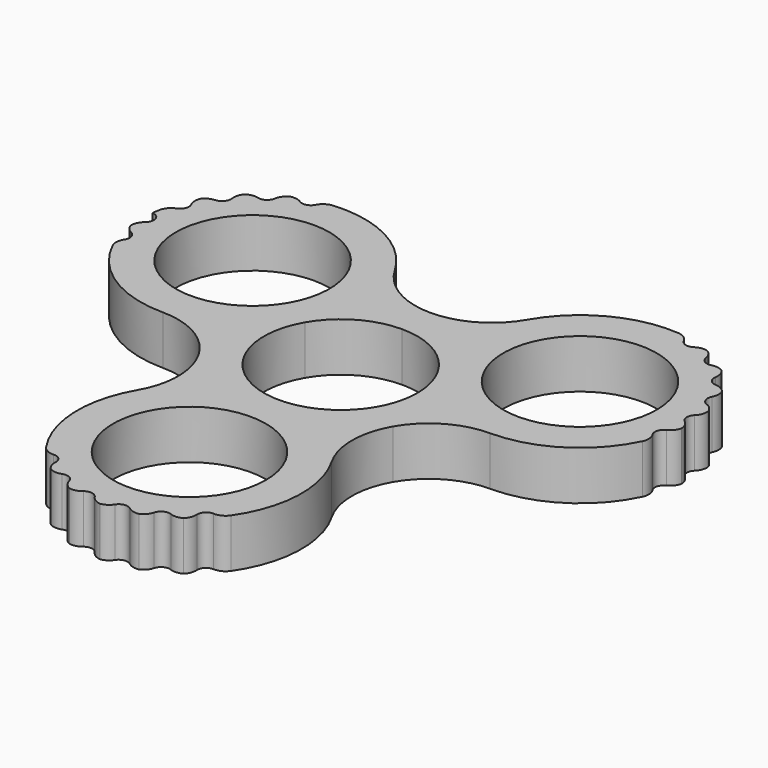
from build123d import *

# Parameters (mm, degrees)
F0_R        = 10.9363137741
F1_DEPTH    = 7.00024
F3_DEPTH    = 7.00124
F4_T1_DEPTH = 14.8104657411
F4_T3_DEPTH = 14.8131793158


# Not quite as in the source:
# - a fillet or chamfer that OpenCascade refuses, or shapes differently, is made with other operations: its cross-section is extruded or revolved along the edge and cut away or added


with BuildPart() as f1:
    # F0 (on Top) → F1 (new body)
    with BuildSketch(Plane.XY):
        with BuildLine():
            ThreePointArc((0, 10.99058), (5.49529, 9.5181214823), (9.5181214823, 5.49529))
            Line((9.5181214823, 5.49529), (13.9175305336, 8.03529))
            ThreePointArc((13.9175305336, 8.03529), (17.9403620159, 23.0487014823), (32.9537734982, 19.02587))
            Line((32.9537734982, 19.02587), (37.3531825494, 21.56587))
            ThreePointArc((37.3531825494, 21.56587), (23.4356520159, 29.60116), (9.5181214823, 21.56587))
            ThreePointArc((9.5181214823, 21.56587), (5.49529, 17.5430385177), (0, 16.07058))
            Line((0, 16.07058), (0, 10.99058))
        make_face()
        with BuildLine():
            Line((13.9175305336, 8.03529), (9.5181214823, 5.49529))
            ThreePointArc((9.5181214823, 5.49529), (10.99058, 0), (9.5181214823, -5.49529))
            Line((9.5181214823, -5.49529), (13.9175305336, -8.03529))
            ThreePointArc((13.9175305336, -8.03529), (17.9403620159, -4.0124585177), (23.4356520159, -2.54))
            ThreePointArc((23.4356520159, -2.54), (37.3531825494, 5.49529), (37.3531825494, 21.56587))
            Line((37.3531825494, 21.56587), (32.9537734982, 19.02587))
            ThreePointArc((32.9537734982, 19.02587), (28.9309420159, 4.0124585177), (13.9175305336, 8.03529))
        make_face()
        with BuildLine():
            Line((13.9175305336, -8.03529), (9.5181214823, -5.49529))
            ThreePointArc((9.5181214823, -5.49529), (0, -10.99058), (-9.5181214823, -5.49529))
            Line((-9.5181214823, -5.49529), (-13.9175305336, -8.03529))
            ThreePointArc((-13.9175305336, -8.03529), (-12.4450720159, -13.53058), (-13.9175305336, -19.02587))
            ThreePointArc((-13.9175305336, -19.02587), (-13.9175305336, -35.09645), (0, -43.13174))
            ThreePointArc((0, -43.13174), (13.9175305336, -35.09645), (13.9175305336, -19.02587))
            ThreePointArc((13.9175305336, -19.02587), (12.4450720159, -13.53058), (13.9175305336, -8.03529))
        make_face()
        with Locations((0, -27.06116)):
            Circle(F0_R, mode=Mode.SUBTRACT)
        with BuildLine():
            ThreePointArc((-9.5181214823, 5.49529), (-5.49529, 9.5181214823), (0, 10.99058))
            Line((0, 10.99058), (0, 16.07058))
            ThreePointArc((0, 16.07058), (-5.49529, 17.5430385177), (-9.5181214823, 21.56587))
            ThreePointArc((-9.5181214823, 21.56587), (-23.4356520159, 29.60116), (-37.3531825494, 21.56587))
            Line((-37.3531825494, 21.56587), (-32.9537734982, 19.02587))
            ThreePointArc((-32.9537734982, 19.02587), (-17.9403620159, 23.0487014823), (-13.9175305336, 8.03529))
            Line((-13.9175305336, 8.03529), (-9.5181214823, 5.49529))
        make_face()
        with BuildLine():
            Line((-13.9175305336, -8.03529), (-9.5181214823, -5.49529))
            ThreePointArc((-9.5181214823, -5.49529), (-10.99058, 0), (-9.5181214823, 5.49529))
            Line((-9.5181214823, 5.49529), (-13.9175305336, 8.03529))
            ThreePointArc((-13.9175305336, 8.03529), (-28.9309420159, 4.0124585177), (-32.9537734982, 19.02587))
            Line((-32.9537734982, 19.02587), (-37.3531825494, 21.56587))
            ThreePointArc((-37.3531825494, 21.56587), (-37.3531825494, 5.49529), (-23.4356520159, -2.54))
            ThreePointArc((-23.4356520159, -2.54), (-17.9403620159, -4.0124585177), (-13.9175305336, -8.03529))
        make_face()
    extrude(amount=F1_DEPTH)

    # F2 (on face) → F3 (cut, through all)
    with BuildSketch(Plane.XY.offset(7.00024)):
        with BuildLine():
            ThreePointArc((-35.0746224958, 24.6120017365), (-35.9139467032, 23.6575589786), (-36.6752197739, 22.6397724514))
            ThreePointArc((-36.6752197739, 22.6397724514), (-34.8888064923, 22.8255884549), (-35.0746224958, 24.6120017365))
        make_face()
        with BuildLine():
            ThreePointArc((-37.9442279658, 20.4417857879), (-38.4450204186, 19.2736107058), (-38.8519299897, 18.0695132413))
            ThreePointArc((-38.8519299897, 18.0695132413), (-37.2119427044, 18.8017985026), (-37.9442279658, 20.4417857879))
        make_face()
        with BuildLine():
            ThreePointArc((-39.3814291193, 15.5295132413), (-39.4895877236, 14.2618048815), (-39.4971210738, 12.9895132413))
            ThreePointArc((-39.4971210738, 12.9895132413), (-38.1692750966, 14.201667264), (-39.3814291193, 15.5295132413))
        make_face()
        with BuildLine():
            ThreePointArc((-31.0484267333, 27.6836433659), (-32.1430835358, 27.0377698581), (-33.1832757705, 26.3074095236))
            ThreePointArc((-33.1832757705, 26.3074095236), (-31.4277343308, 25.9281019262), (-31.0484267333, 27.6836433659))
        make_face()
        with BuildLine():
            ThreePointArc((-39.2112581719, 10.4656506457), (-38.9197100236, 9.2285468584), (-38.5313098328, 8.0183520828))
            ThreePointArc((-38.5313098328, 8.0183520828), (-37.6476347209, 9.5819755338), (-39.2112581719, 10.4656506457))
        make_face()
        with BuildLine():
            ThreePointArc((-26.2662923178, 29.3499041644), (-27.507583715, 29.0767343082), (-28.7234053742, 28.7063240001))
            ThreePointArc((-28.7234053742, 28.7063240001), (-27.1730587639, 27.799557554), (-26.2662923178, 29.3499041644))
        make_face()
        with BuildLine():
            ThreePointArc((26.2662923178, 29.3499041644), (27.1730587639, 27.799557554), (28.7234053742, 28.7063240001))
            ThreePointArc((28.7234053742, 28.7063240001), (27.507583715, 29.0767343082), (26.2662923178, 29.3499041644))
        make_face()
        with BuildLine():
            ThreePointArc((31.0484267333, 27.6836433659), (31.4277343308, 25.9281019262), (33.1832757705, 26.3074095236))
            ThreePointArc((33.1832757705, 26.3074095236), (32.1430835358, 27.0377698581), (31.0484267333, 27.6836433659))
        make_face()
        with BuildLine():
            ThreePointArc((35.0746224958, 24.6120017365), (34.8888064923, 22.8255884549), (36.6752197739, 22.6397724514))
            ThreePointArc((36.6752197739, 22.6397724514), (35.9139467032, 23.6575589786), (35.0746224958, 24.6120017365))
        make_face()
        with BuildLine():
            ThreePointArc((37.9442279658, 20.4417857879), (37.2119427044, 18.8017985026), (38.8519299897, 18.0695132413))
            ThreePointArc((38.8519299897, 18.0695132413), (38.4450204186, 19.2736107058), (37.9442279658, 20.4417857879))
        make_face()
        with BuildLine():
            ThreePointArc((39.3814291193, 15.5295132413), (38.1692750966, 14.201667264), (39.4971210738, 12.9895132413))
            ThreePointArc((39.4971210738, 12.9895132413), (39.4895877236, 14.2618048815), (39.3814291193, 15.5295132413))
        make_face()
        with BuildLine():
            ThreePointArc((39.2112581719, 10.4656506457), (37.6476347209, 9.5819755338), (38.5313098328, 8.0183520828))
            ThreePointArc((38.5313098328, 8.0183520828), (38.9197100236, 9.2285468584), (39.2112581719, 10.4656506457))
        make_face()
        with BuildLine():
            ThreePointArc((1.2690081918, -43.0815582393), (2.5310737154, -42.9311696844), (3.7773074939, -42.6815149778))
            ThreePointArc((3.7773074939, -42.6815149778), (2.3231362121, -41.6273869575), (1.2690081918, -43.0815582393))
        make_face()
        with BuildLine():
            ThreePointArc((6.19124707, -41.8912645598), (7.3438537909, -41.355611827), (8.4505250575, -40.7305479815))
            ThreePointArc((8.4505250575, -40.7305479815), (6.7405277746, -40.1812672769), (6.19124707, -41.8912645598))
        make_face()
        with BuildLine():
            ThreePointArc((10.4987031463, -39.2283607373), (11.4273987125, -38.360633448), (12.2846164461, -37.4222284926))
            ThreePointArc((12.2846164461, -37.4222284926), (10.4885936738, -37.432337965), (10.4987031463, -39.2283607373))
        make_face()
        with BuildLine():
            ThreePointArc((-3.7773074939, -42.6815149778), (-2.5310737154, -42.9311696844), (-1.2690081918, -43.0815582393))
            ThreePointArc((-1.2690081918, -43.0815582393), (-2.3231362121, -41.6273869575), (-3.7773074939, -42.6815149778))
        make_face()
        with BuildLine():
            ThreePointArc((-8.4505250575, -40.7305479815), (-7.3438537909, -41.355611827), (-6.19124707, -41.8912645598))
            ThreePointArc((-6.19124707, -41.8912645598), (-6.7405277746, -40.1812672769), (-8.4505250575, -40.7305479815))
        make_face()
        with BuildLine():
            ThreePointArc((-12.2846164461, -37.4222284926), (-11.4273987125, -38.360633448), (-10.4987031463, -39.2283607373))
            ThreePointArc((-10.4987031463, -39.2283607373), (-10.4885936738, -37.432337965), (-12.2846164461, -37.4222284926))
        make_face()
    extrude(amount=-F3_DEPTH, mode=Mode.SUBTRACT)

    # F4: fillet of radius 2.032 on 35 edges, made by hand

    # F4_s2 → F4_t1 (cut)
    with BuildSketch(Plane.XY.offset(-3.9051128705)):
        with BuildLine():
            ThreePointArc((6.0917538688, -40.991322092), (5.5931519946, -41.8849684391), (4.7222318964, -42.4222819464))
            ThreePointArc((4.7222318964, -42.4222819464), (5.4631950957, -42.174632165), (6.19124707, -41.8912645598))
            ThreePointArc((6.19124707, -41.8912645598), (6.0585768736, -41.4504609497), (6.0917538688, -40.991322092))
        make_face()
        with BuildLine():
            ThreePointArc((13.2324820436, -36.180642469), (12.4583166764, -36.8498775598), (11.4561512142, -37.0569331298))
            ThreePointArc((11.4561512142, -37.0569331298), (11.9040433207, -37.163243358), (12.2846164461, -37.4222284926))
            ThreePointArc((12.2846164461, -37.4222284926), (12.773643286, -36.8129587438), (13.2324820436, -36.180642469))
        make_face()
        with BuildLine():
            ThreePointArc((1.4544998037, -42.1953369326), (0.7025673824, -42.8894588646), (-0.2923138781, -43.129081276))
            ThreePointArc((-0.2923138781, -43.129081276), (0.4889248975, -43.1243008504), (1.2690081918, -43.0815582393))
            ThreePointArc((1.2690081918, -43.0815582393), (1.2800947139, -42.6213557917), (1.4544998037, -42.1953369326))
        make_face()
        with BuildLine():
            ThreePointArc((9.7376877828, -39.8455637085), (8.793705947, -40.2406661209), (7.7768655807, -40.1255866175))
            ThreePointArc((7.7768655807, -40.1255866175), (8.1694384065, -40.3659941469), (8.4505250575, -40.7305479815))
            ThreePointArc((8.4505250575, -40.7305479815), (9.1048652309, -40.303703965), (9.7376877828, -39.8455637085))
        make_face()
        with BuildLine():
            ThreePointArc((5.2759537583, -42.2410102455), (4.2558916256, -42.3227468226), (3.3253472844, -41.8969594912))
            ThreePointArc((3.3253472844, -41.8969594912), (3.6236188571, -42.247592166), (3.7773074939, -42.6815149778))
            ThreePointArc((3.7773074939, -42.6815149778), (4.5319858705, -42.4794817506), (5.2759537583, -42.2410102455))
        make_face()
        with BuildLine():
            ThreePointArc((-3.3253472844, -41.8969594912), (-4.2558916256, -42.3227468226), (-5.2759537583, -42.2410102455))
            ThreePointArc((-5.2759537583, -42.2410102455), (-4.5319858705, -42.4794817506), (-3.7773074939, -42.6815149778))
            ThreePointArc((-3.7773074939, -42.6815149778), (-3.6236188571, -42.247592166), (-3.3253472844, -41.8969594912))
        make_face()
        with BuildLine():
            ThreePointArc((0.2923138781, -43.129081276), (-0.7025673824, -42.8894588646), (-1.4544998037, -42.1953369326))
            ThreePointArc((-1.4544998037, -42.1953369326), (-1.2800947139, -42.6213557917), (-1.2690081918, -43.0815582393))
            ThreePointArc((-1.2690081918, -43.0815582393), (-0.4889248975, -43.1243008504), (0.2923138781, -43.129081276))
        make_face()
        with BuildLine():
            ThreePointArc((-7.7768655807, -40.1255866175), (-8.793705947, -40.2406661209), (-9.7376877828, -39.8455637085))
            ThreePointArc((-9.7376877828, -39.8455637085), (-9.1048652309, -40.303703965), (-8.4505250575, -40.7305479815))
            ThreePointArc((-8.4505250575, -40.7305479815), (-8.1694384065, -40.3659941469), (-7.7768655807, -40.1255866175))
        make_face()
        with BuildLine():
            ThreePointArc((-4.7222318964, -42.4222819464), (-5.5931519946, -41.8849684391), (-6.0917538688, -40.991322092))
            ThreePointArc((-6.0917538688, -40.991322092), (-6.0585768736, -41.4504609497), (-6.19124707, -41.8912645598))
            ThreePointArc((-6.19124707, -41.8912645598), (-5.4631950957, -42.174632165), (-4.7222318964, -42.4222819464))
        make_face()
        with BuildLine():
            ThreePointArc((-11.4561512142, -37.0569331298), (-12.4583166764, -36.8498775598), (-13.2324820436, -36.180642469))
            ThreePointArc((-13.2324820436, -36.180642469), (-12.773643286, -36.8129587438), (-12.2846164461, -37.4222284926))
            ThreePointArc((-12.2846164461, -37.4222284926), (-11.9040433207, -37.163243358), (-11.4561512142, -37.0569331298))
        make_face()
        with BuildLine():
            ThreePointArc((-26.3641698697, 28.449784546), (-25.6837717549, 29.21415751), (-24.7171144815, 29.5499868394))
            ThreePointArc((-24.7171144815, 29.5499868394), (-25.4941358176, 29.4687789564), (-26.2662923178, 29.3499041644))
            ThreePointArc((-26.2662923178, 29.3499041644), (-26.2322911747, 28.8908256025), (-26.3641698697, 28.449784546))
        make_face()
        with BuildLine():
            ThreePointArc((-34.3776579039, 25.3007137581), (-33.4768707076, 25.7862959341), (-32.453649332, 25.7712746499))
            ThreePointArc((-32.453649332, 25.7712746499), (-32.8678637442, 25.9721119581), (-33.1832757705, 26.3074095236))
            ThreePointArc((-33.1832757705, 26.3074095236), (-33.7927053023, 25.8185818212), (-34.3776579039, 25.3007137581))
        make_face()
        with BuildLine():
            ThreePointArc((-30.8613445622, 26.7977564635), (-30.4525861524, 27.735905804), (-29.6384265082, 28.3558668483))
            ThreePointArc((-29.6384265082, 28.3558668483), (-30.3515988849, 28.0368965704), (-31.0484267333, 27.6836433659))
            ThreePointArc((-31.0484267333, 27.6836433659), (-30.873257177, 27.2579382681), (-30.8613445622, 26.7977564635))
        make_face()
        with BuildLine():
            ThreePointArc((-37.497036966, 21.3113893937), (-36.7920772401, 22.0531706333), (-35.814983803, 22.3573022461))
            ThreePointArc((-35.814983803, 22.3573022461), (-36.2711295024, 22.4192724374), (-36.6752197739, 22.6397724514))
            ThreePointArc((-36.6752197739, 22.6397724514), (-37.1022776082, 21.985571807), (-37.497036966, 21.3113893937))
        make_face()
        with BuildLine():
            ThreePointArc((-34.6211576186, 23.8283149703), (-34.5246280935, 24.8470836749), (-33.943811075, 25.6896151067))
            ThreePointArc((-33.943811075, 25.6896151067), (-34.5223174004, 25.1645557687), (-35.0746224958, 24.6120017365))
            ThreePointArc((-35.0746224958, 24.6120017365), (-34.775678636, 24.2619420669), (-34.6211576186, 23.8283149703))
        make_face()
        with BuildLine():
            ThreePointArc((-39.2197648333, 16.5513951388), (-38.7805197191, 17.4756631478), (-37.9465049029, 18.0686445209))
            ThreePointArc((-37.9465049029, 18.0686445209), (-38.399297493, 17.9856500992), (-38.8519299897, 18.0695132413))
            ThreePointArc((-38.8519299897, 18.0695132413), (-39.0543032709, 17.3149259819), (-39.2197648333, 16.5513951388))
        make_face()
        with BuildLine():
            ThreePointArc((-37.2694836067, 19.8380346865), (-37.4946446225, 20.8362882312), (-37.2047230879, 21.8176918823))
            ThreePointArc((-37.2047230879, 21.8176918823), (-37.5912025057, 21.1387290435), (-37.9442279658, 20.4417857879))
            ThreePointArc((-37.9442279658, 20.4417857879), (-37.5512242163, 20.2020833544), (-37.2694836067, 19.8380346865))
        make_face()
        with BuildLine():
            ThreePointArc((-37.924850324, 6.5788410862), (-38.1209321148, 7.5832113137), (-37.8026377531, 8.5557833275))
            ThreePointArc((-37.8026377531, 8.5557833275), (-38.1174531481, 8.2199255142), (-38.5313098328, 8.0183520828))
            ThreePointArc((-38.5313098328, 8.0183520828), (-38.2455803061, 7.2912238173), (-37.924850324, 6.5788410862))
        make_face()
        with BuildLine():
            ThreePointArc((-38.3097860173, 10.3811326178), (-39.0841652168, 11.0501202694), (-39.4342931277, 12.0116908953))
            ThreePointArc((-39.4342931277, 12.0116908953), (-39.3415709605, 11.2359593202), (-39.2112581719, 10.4656506457))
            ThreePointArc((-39.2112581719, 10.4656506457), (-38.7527343314, 10.5064561778), (-38.3097860173, 10.3811326178))
        make_face()
        with BuildLine():
            ThreePointArc((-30.1717518527, 28.1212791102), (-29.1645841861, 28.3024445425), (-28.1968394269, 27.9697619555))
            ThreePointArc((-28.1968394269, 27.9697619555), (-28.5279915983, 28.2895234965), (-28.7234053742, 28.7063240001))
            ThreePointArc((-28.7234053742, 28.7063240001), (-29.4546910418, 28.4314091964), (-30.1717518527, 28.1212791102))
        make_face()
        with BuildLine():
            ThreePointArc((-9.26786617, -40.1901431362), (-9.92834387, -39.4084930672), (-10.1241046778, -38.4040602278))
            ThreePointArc((-10.1241046778, -38.4040602278), (-10.2354502098, -38.8507271913), (-10.4987031463, -39.2283607373))
            ThreePointArc((-10.4987031463, -39.2283607373), (-9.8949771086, -39.724215301), (-9.26786617, -40.1901431362))
        make_face()
        with BuildLine():
            ThreePointArc((10.1241046778, -38.4040602278), (9.92834387, -39.4084930672), (9.26786617, -40.1901431362))
            ThreePointArc((9.26786617, -40.1901431362), (9.8949771086, -39.724215301), (10.4987031463, -39.2283607373))
            ThreePointArc((10.4987031463, -39.2283607373), (10.2354502098, -38.8507271913), (10.1241046778, -38.4040602278))
        make_face()
        with BuildLine():
            ThreePointArc((24.7171144815, 29.5499868394), (25.6837717549, 29.21415751), (26.3641698697, 28.449784546))
            ThreePointArc((26.3641698697, 28.449784546), (26.2322911747, 28.8908256025), (26.2662923178, 29.3499041644))
            ThreePointArc((26.2662923178, 29.3499041644), (25.4941358176, 29.4687789564), (24.7171144815, 29.5499868394))
        make_face()
        with BuildLine():
            ThreePointArc((28.1968394269, 27.9697619555), (29.1645841861, 28.3024445425), (30.1717518527, 28.1212791102))
            ThreePointArc((30.1717518527, 28.1212791102), (29.4546910418, 28.4314091964), (28.7234053742, 28.7063240001))
            ThreePointArc((28.7234053742, 28.7063240001), (28.5279915983, 28.2895234965), (28.1968394269, 27.9697619555))
        make_face()
        with BuildLine():
            ThreePointArc((29.6384265082, 28.3558668483), (30.4525861524, 27.735905804), (30.8613445622, 26.7977564635))
            ThreePointArc((30.8613445622, 26.7977564635), (30.873257177, 27.2579382681), (31.0484267333, 27.6836433659))
            ThreePointArc((31.0484267333, 27.6836433659), (30.3515988849, 28.0368965704), (29.6384265082, 28.3558668483))
        make_face()
        with BuildLine():
            ThreePointArc((32.453649332, 25.7712746499), (33.4768707076, 25.7862959341), (34.3776579039, 25.3007137581))
            ThreePointArc((34.3776579039, 25.3007137581), (33.7927053023, 25.8185818212), (33.1832757705, 26.3074095236))
            ThreePointArc((33.1832757705, 26.3074095236), (32.8678637442, 25.9721119581), (32.453649332, 25.7712746499))
        make_face()
        with BuildLine():
            ThreePointArc((33.943811075, 25.6896151067), (34.5246280935, 24.8470836749), (34.6211576185, 23.8283149703))
            ThreePointArc((34.6211576185, 23.8283149703), (34.775678636, 24.2619420669), (35.0746224958, 24.6120017365))
            ThreePointArc((35.0746224958, 24.6120017365), (34.5223174004, 25.1645557687), (33.943811075, 25.6896151067))
        make_face()
        with BuildLine():
            ThreePointArc((35.814983803, 22.3573022461), (36.7920772401, 22.0531706333), (37.497036966, 21.3113893937))
            ThreePointArc((37.497036966, 21.3113893937), (37.1022776082, 21.985571807), (36.6752197739, 22.6397724514))
            ThreePointArc((36.6752197739, 22.6397724514), (36.2711295024, 22.4192724374), (35.814983803, 22.3573022461))
        make_face()
        with BuildLine():
            ThreePointArc((37.2047230879, 21.8176918823), (37.4946446225, 20.8362882312), (37.2694836067, 19.8380346865))
            ThreePointArc((37.2694836067, 19.8380346865), (37.5512242163, 20.2020833544), (37.9442279658, 20.4417857879))
            ThreePointArc((37.9442279658, 20.4417857879), (37.5912025057, 21.1387290435), (37.2047230879, 21.8176918823))
        make_face()
        with BuildLine():
            ThreePointArc((37.9465049029, 18.0686445209), (38.7805197191, 17.4756631478), (39.2197648333, 16.5513951388))
            ThreePointArc((39.2197648333, 16.5513951388), (39.0543032709, 17.3149259819), (38.8519299897, 18.0695132413))
            ThreePointArc((38.8519299897, 18.0695132413), (38.399297493, 17.9856500992), (37.9465049029, 18.0686445209))
        make_face()
        with BuildLine():
            ThreePointArc((37.8026377531, 8.5557833275), (38.1209321148, 7.5832113137), (37.924850324, 6.5788410862))
            ThreePointArc((37.924850324, 6.5788410862), (38.2455803061, 7.2912238173), (38.5313098328, 8.0183520828))
            ThreePointArc((38.5313098328, 8.0183520828), (38.1174531481, 8.2199255142), (37.8026377531, 8.5557833275))
        make_face()
        with BuildLine():
            ThreePointArc((39.4342931277, 12.0116908953), (39.0841652168, 11.0501202694), (38.3097860173, 10.3811326178))
            ThreePointArc((38.3097860173, 10.3811326178), (38.7527343314, 10.5064561778), (39.2112581719, 10.4656506457))
            ThreePointArc((39.2112581719, 10.4656506457), (39.3415709605, 11.2359593202), (39.4342931277, 12.0116908953))
        make_face()
    extrude(amount=F4_T1_DEPTH, mode=Mode.SUBTRACT)

    # F4_s4 → F4_t3 (cut)
    with BuildSketch(Plane.XY.offset(-3.9064696579)):
        with BuildLine():
            ThreePointArc((39.1119195679, 17.0686836125), (39.0784858979, 16.0455064211), (38.5504402165, 15.1684789794))
            ThreePointArc((38.5504402165, 15.1684789794), (38.932680983, 15.4255357801), (39.3814291193, 15.5295132413))
            ThreePointArc((39.3814291193, 15.5295132413), (39.2653926457, 16.3023760115), (39.1119195679, 17.0686836125))
        make_face()
        with BuildLine():
            ThreePointArc((38.6367523111, 13.2735095213), (39.2423398483, 12.4481168207), (39.3686494886, 11.4322156198))
            ThreePointArc((39.3686494886, 11.4322156198), (39.451824034, 12.2093020499), (39.4971210738, 12.9895132413))
            ThreePointArc((39.4971210738, 12.9895132413), (39.040778724, 13.0522656287), (38.6367523111, 13.2735095213))
        make_face()
        with BuildLine():
            ThreePointArc((-39.3686494886, 11.4322156198), (-39.2423398483, 12.4481168207), (-38.6367523111, 13.2735095212))
            ThreePointArc((-38.6367523111, 13.2735095212), (-39.040778724, 13.0522656287), (-39.4971210738, 12.9895132413))
            ThreePointArc((-39.4971210738, 12.9895132413), (-39.451824034, 12.2093020499), (-39.3686494886, 11.4322156198))
        make_face()
    extrude(amount=F4_T3_DEPTH, mode=Mode.SUBTRACT)


solid = f1.part
